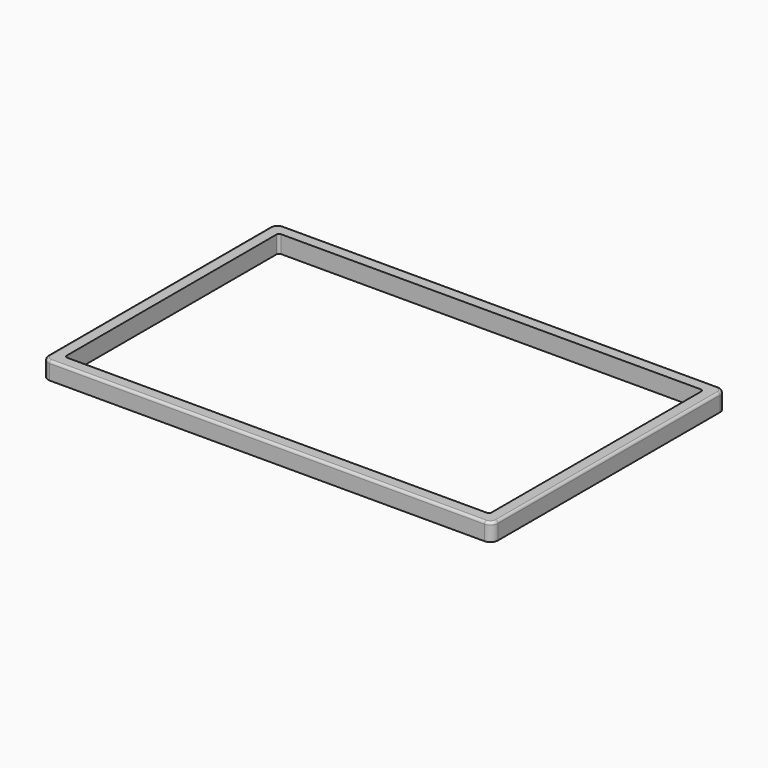
from build123d import *

# Parameters (mm, degrees)
F0_W     = 180
F0_H     = 117
F2_DEPTH = 7
F1_W     = 170
F1_H     = 107
F3_DEPTH = 25
F4_R     = 3
F5_R     = 1
F6_R     = 1


with BuildPart() as f2:
    # F0 (on Top) → F2 (new body)
    with BuildSketch(Plane.XY):
        with Locations((-29.744874835, 27.1624445021)):
            Rectangle(F0_W, F0_H)
    extrude(amount=F2_DEPTH)

    # F1 (on face) → F3 (cut)
    with BuildSketch(Plane.XY):
        with Locations((-29.744874835, 27.1624445021)):
            Rectangle(F1_W, F1_H)
    extrude(amount=F3_DEPTH, mode=Mode.SUBTRACT)

    # F4
    f4_edges = [f2.edges().sort_by_distance(p)[0] for p in [
        (60.255125, 85.662445, 3.5),
        (60.255125, -31.337555, 3.5),
        (-119.744875, -31.337555, 3.5),
        (-119.744875, 85.662445, 3.5),
    ]]
    fillet(f4_edges, radius=F4_R)

    # F5
    f5_edges = [f2.edges().sort_by_distance(p)[0] for p in [
        (-119.744875, 27.162445, 7),
        (-29.744875, -31.337555, 7),
        (-118.866195, -30.458876, 7),
    ]]
    fillet(f5_edges, radius=F5_R)

    # F6
    f6_edges = [f2.edges().sort_by_distance(p)[0] for p in [
        (55.255125, -26.337555, 3.5),
        (55.255125, 80.662445, 3.5),
        (-114.744875, 80.662445, 3.5),
        (-114.744875, -26.337555, 3.5),
    ]]
    fillet(f6_edges, radius=F6_R)


solid = f2.part
